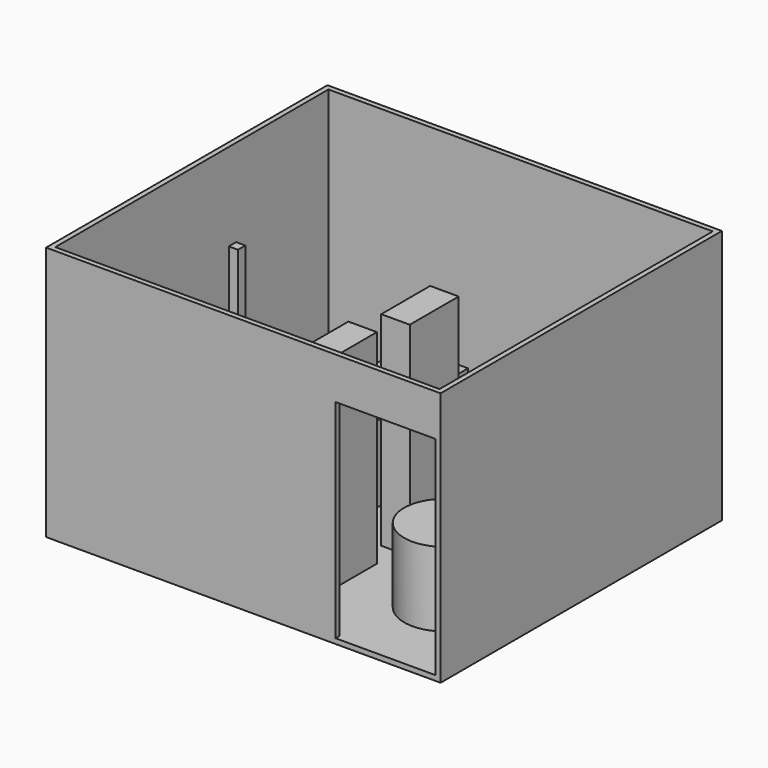
from build123d import *

# Parameters (mm, degrees)
F0_W      = 387
F0_H      = 345
F1_DEPTH  = 250
F2_W      = 377
F2_H      = 335
F3_DEPTH  = 245
F4_W      = 98
F4_H      = 204
F5_DEPTH  = 25
F6_W      = 9
F6_H      = 9
F7_DEPTH  = 245
F8_W      = 60
F8_H      = 120
F9_DEPTH  = 75
F10_W     = 120
F10_H     = 23.8507700859
F11_DEPTH = 75
F12_W     = 28
F12_H     = 60
F13_DEPTH = 200
F14_W     = 28
F14_H     = 60
F15_DEPTH = 200
F16_R     = 40
F17_DEPTH = 73
F18_W     = 66
F18_H     = 92
F18_W_2   = 9
F18_H_2   = 9
F19_DEPTH = 147


with BuildPart() as f1:
    # F0 (on Top) → F1 (new body)
    with BuildSketch(Plane.XY):
        with Locations((-193.5, 172.5)):
            Rectangle(F0_W, F0_H)
    extrude(amount=F1_DEPTH)

    # F2 (on face) → F3 (cut)
    with BuildSketch(Plane.XY.offset(250)):
        with Locations((-193.5, 172.5)):
            Rectangle(F2_W, F2_H)
    extrude(amount=-F3_DEPTH, mode=Mode.SUBTRACT)

    # F4 (on face) → F5 (cut)
    with BuildSketch(Plane(origin=(0, 5, 0), x_dir=(-1, 0, 0), z_dir=(0, 1, 0))):
        with Locations((54, 107)):
            Rectangle(F4_W, F4_H)
    extrude(amount=-F5_DEPTH, mode=Mode.SUBTRACT)

    # F6 (on face) → F7 (join)
    with BuildSketch(Plane.XY.offset(5)):
        with Locations((-274.5, 93.5)):
            Rectangle(F6_W, F6_H)
    extrude(amount=F7_DEPTH)

    # F8 (on face) → F9 (join)
    with BuildSketch(Plane.XY.offset(5)):
        with Locations((-243.4864774462, 240.5474260449)):
            Rectangle(F8_W, F8_H)
    extrude(amount=F9_DEPTH)

    # F10 (on face) → F11 (join)
    with BuildSketch(Plane.XY.offset(5)):
        with Locations((-110.3469633506, 351.925385043)):
            Rectangle(F10_W, F10_H)
    extrude(amount=F11_DEPTH)

    # F14 (on face) → F15 (join)
    with BuildSketch(Plane.XY.offset(5)):
        with Locations((-169.5094383758, 86.3268319517)):
            Rectangle(F14_W, F14_H)
    extrude(amount=F15_DEPTH)

    # F16 (on face) → F17 (join)
    with BuildSketch(Plane.XY.offset(5)):
        with Locations((-69.5516467094, 92.2992378473)):
            Circle(F16_R)
    extrude(amount=F17_DEPTH)

    # F18 (on face) → F19 (join)
    with BuildSketch(Plane.XY.offset(5)):
        with Locations((-279.4643215769, 66.0552727059)):
            Rectangle(F18_W, F18_H)
        with Locations((-274.5, 93.5)):
            Rectangle(F18_W_2, F18_H_2, mode=Mode.SUBTRACT)
    extrude(amount=F19_DEPTH)


with BuildPart() as f13:
    # F12 (on face) → F13 (new body)
    with BuildSketch(Plane.XY.offset(5)):
        with Locations((-157.5231286956, 171.648837626)):
            Rectangle(F12_W, F12_H)
    extrude(amount=F13_DEPTH)


solid = Compound([f1.part, f13.part])
